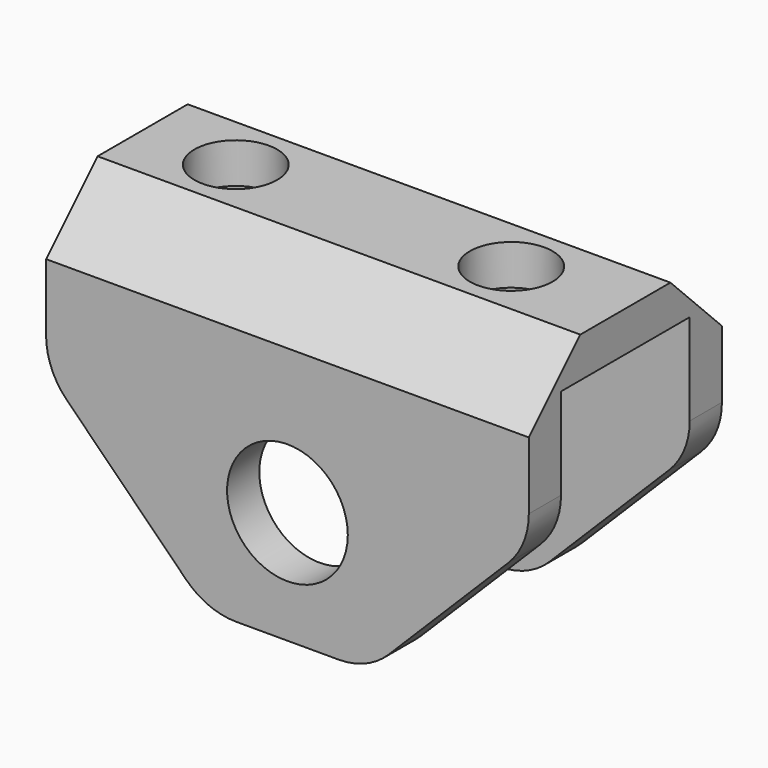
from build123d import *

# Parameters (mm, degrees)
F0_W        = 38.1
F0_H        = 19.05
F1_DEPTH    = 25.4
F2_R        = 3.2639
F3_DEPTH    = 25.4
F4_R        = 4.7625
F5_DEPTH    = 25.4
F6_T1_DEPTH = 84.3707478943
F7_W        = 12.7
F7_H        = 22.225
F8_DEPTH    = 38.1
F9_R        = 5.588
F10_SIZE    = 5.08


# Not quite as in the source:
# - a fillet or chamfer that OpenCascade refuses, or shapes differently, is made with other operations: its cross-section is extruded or revolved along the edge and cut away or added


with BuildPart() as f1:
    # F0 (on Top) → F1 (new body)
    with BuildSketch(Plane.XY):
        with Locations((19.05, 9.525)):
            Rectangle(F0_W, F0_H)
    extrude(amount=-F1_DEPTH)

    # F2 (on face) → F3 (cut)
    with BuildSketch(Plane.XY):
        with Locations((7.3534409022, 9.525)):
            Circle(F2_R)
        with Locations((29.0893973289, 9.525)):
            Circle(F2_R)
    extrude(amount=-F3_DEPTH, mode=Mode.SUBTRACT)

    # F4 (on face) → F5 (cut)
    with BuildSketch(Plane.XZ):
        with Locations((19.05, -16.51)):
            Circle(F4_R)
    extrude(amount=-F5_DEPTH, mode=Mode.SUBTRACT)

    # F6: chamfer of 12.7 on 2 edges, made by hand

    # F6_s2 → F6_t1 (cut)
    with BuildSketch(Plane.XZ.offset(-51.7103739472)):
        Polygon((25.4, -25.4), (38.1, -12.7), (38.1, -25.4), align=None)
        Polygon((0, -12.7), (12.7, -25.4), (0, -25.4), align=None)
    extrude(amount=F6_T1_DEPTH, mode=Mode.SUBTRACT)

    # F7 (on Right) → F8 (cut)
    with BuildSketch(Plane.YZ):
        with Locations((9.525, -14.2875)):
            Rectangle(F7_W, F7_H)
    extrude(amount=F8_DEPTH, mode=Mode.SUBTRACT)

    # F9
    f9_edges = [f1.edges().sort_by_distance(p)[0] for p in [
        (0, 17.4625, -12.7),
        (0, 1.5875, -12.7),
        (12.7, 17.4625, -25.4),
        (12.7, 1.5875, -25.4),
        (25.4, 1.5875, -25.4),
        (25.4, 17.4625, -25.4),
        (38.1, 17.4625, -12.7),
        (38.1, 1.5875, -12.7),
    ]]
    fillet(f9_edges, radius=F9_R)

    # F10
    f10_edges = [f1.edges().sort_by_distance(p)[0] for p in [
        (19.05, 19.05, 0),
        (19.05, 0, 0),
    ]]
    chamfer(f10_edges, length=F10_SIZE)


solid = f1.part
